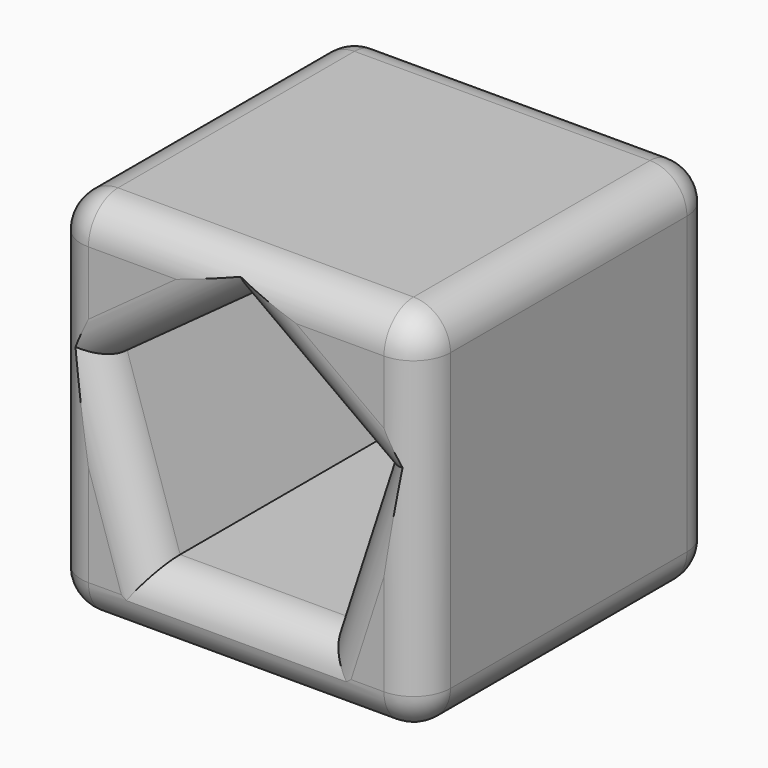
from build123d import *

# Parameters (mm, degrees)
F0_W          = 100
F0_H          = 100
F1_DEPTH      = 100
F3_DEPTH      = 134.3
F4_T1_DEPTH   = 80
F4_T3_DEPTH   = 80
F4_T5_DEPTH   = 80
F4_S9_W       = 10
F4_S9_H       = 10
F4_T10_DEPTH  = 10
F4_S15_W      = 10
F4_S15_H      = 10
F4_T16_DEPTH  = 10
F4_S21_W      = 10
F4_S21_H      = 10
F4_T22_DEPTH  = 10
F4_S27_W      = 10
F4_S27_H      = 10
F4_T28_DEPTH  = 10
F4_S33_W      = 10
F4_S33_H      = 10
F4_T34_DEPTH  = 10
F4_S39_W      = 10
F4_S39_H      = 10
F4_T40_DEPTH  = 10
F4_S45_W      = 10
F4_S45_H      = 10
F4_T46_DEPTH  = 10
F4_S51_W      = 10
F4_S51_H      = 10
F4_T52_DEPTH  = 10
F4_T58_DEPTH  = 96.3793887771
F4_T64_DEPTH  = 96.3793887771
F4_T70_DEPTH  = 96.3793887771
F4_T76_DEPTH  = 96.3793887771
F4_T82_DEPTH  = 96.3793887771
F4_T88_DEPTH  = 96.3793887771
F4_T94_DEPTH  = 96.3793887771
F4_T100_DEPTH = 96.3793887771
F4_T106_DEPTH = 96.3793887771
F4_T112_DEPTH = 96.3793887771
F4_T119_DEPTH = 96.3793887771
F4_T123_DEPTH = 96.3793887771
F4_T130_DEPTH = 96.3793887771
F4_T134_DEPTH = 96.3793887771
F4_T141_DEPTH = 96.3793887771
F4_T145_DEPTH = 96.3793887771
F4_T152_DEPTH = 96.3793887771
F4_T156_DEPTH = 96.3793887771
F4_T163_DEPTH = 96.3793887771
F4_T167_DEPTH = 96.3793887771
F4_T174_DEPTH = 96.3793887771
F4_T178_DEPTH = 96.3793887771
F4_T185_DEPTH = 96.3793887771
F4_T189_DEPTH = 96.3793887771
F4_T196_DEPTH = 96.3793887771
F4_T200_DEPTH = 96.3793887771
F4_T207_DEPTH = 96.3793887771
F4_T211_DEPTH = 96.3793887771
F4_T218_DEPTH = 96.3793887771
F4_T222_DEPTH = 96.3793887771


# Not quite as in the source:
# - a fillet or chamfer that OpenCascade refuses, or shapes differently, is made with other operations: its cross-section is extruded or revolved along the edge and cut away or added


with BuildPart() as f1:
    # F0 (on Front) → F1 (new body)
    with BuildSketch(Plane.XZ):
        Rectangle(F0_W, F0_H)
    extrude(amount=F1_DEPTH)

    # F2 (on face) → F3 (cut)
    with BuildSketch(Plane.XZ.offset(100)):
        Polygon((37.5217137094, 12.1915438206), (0, 39.4526645541), (-37.5217137094, 12.1915438206), (-23.1896943886, -31.9178760977), (23.1896943886, -31.9178760977), align=None)
    extrude(amount=-F3_DEPTH, mode=Mode.SUBTRACT)

    # F4: fillet of radius 10 on 22 edges, made by hand

    # F4_s2 → F4_t1 (cut)
    with BuildSketch(Plane.XZ.offset(10)):
        with BuildLine():
            ThreePointArc((50, -40), (47.0710678119, -47.0710678119), (40, -50))
            Line((40, -50), (50, -50))
            Line((50, -50), (50, -40))
        make_face()
        with BuildLine():
            ThreePointArc((50, 40), (47.0710678119, 47.0710678119), (40, 50))
            Line((40, 50), (50, 50))
            Line((50, 50), (50, 40))
        make_face()
        with BuildLine():
            ThreePointArc((-40, 50), (-47.0710678119, 47.0710678119), (-50, 40))
            Line((-50, 40), (-50, 50))
            Line((-50, 50), (-40, 50))
        make_face()
        with BuildLine():
            ThreePointArc((-40, -50), (-47.0710678119, -47.0710678119), (-50, -40))
            Line((-50, -40), (-50, -50))
            Line((-50, -50), (-40, -50))
        make_face()
    extrude(amount=F4_T1_DEPTH, mode=Mode.SUBTRACT)

    # F4_s4 → F4_t3 (cut)
    with BuildSketch(Plane.XY.offset(-40)):
        with BuildLine():
            ThreePointArc((50, -10), (47.0710678119, -2.9289321881), (40, 0))
            Line((40, 0), (50, 0))
            Line((50, 0), (50, -10))
        make_face()
        with BuildLine():
            ThreePointArc((50, -90), (47.0710678119, -97.0710678119), (40, -100))
            Line((40, -100), (50, -100))
            Line((50, -100), (50, -90))
        make_face()
        with BuildLine():
            ThreePointArc((-40, 0), (-47.0710678119, -2.9289321881), (-50, -10))
            Line((-50, -10), (-50, 0))
            Line((-50, 0), (-40, 0))
        make_face()
        with BuildLine():
            ThreePointArc((-40, -100), (-47.0710678119, -97.0710678119), (-50, -90))
            Line((-50, -90), (-50, -100))
            Line((-50, -100), (-40, -100))
        make_face()
    extrude(amount=F4_T3_DEPTH, mode=Mode.SUBTRACT)

    # F4_s6 → F4_t5 (cut)
    with BuildSketch(Plane.YZ.offset(-40)):
        with BuildLine():
            ThreePointArc((-10, 50), (-2.9289321881, 47.0710678119), (0, 40))
            Line((0, 40), (0, 50))
            Line((0, 50), (-10, 50))
        make_face()
        with BuildLine():
            ThreePointArc((-90, 50), (-97.0710678119, 47.0710678119), (-100, 40))
            Line((-100, 40), (-100, 50))
            Line((-100, 50), (-90, 50))
        make_face()
        with BuildLine():
            ThreePointArc((-10, -50), (-2.9289321881, -47.0710678119), (0, -40))
            Line((0, -40), (0, -50))
            Line((0, -50), (-10, -50))
        make_face()
        with BuildLine():
            ThreePointArc((-90, -50), (-97.0710678119, -47.0710678119), (-100, -40))
            Line((-100, -40), (-100, -50))
            Line((-100, -50), (-90, -50))
        make_face()
    extrude(amount=F4_T5_DEPTH, mode=Mode.SUBTRACT)


with BuildPart() as f4_tool8:
    # F4_s9 → F4_t10 (new body)
    with BuildSketch(Plane.YZ.offset(40)):
        with Locations((-5, -45)):
            Rectangle(F4_S9_W, F4_S9_H)
    extrude(amount=F4_T10_DEPTH)

    # F4_s11 → F4_t12 (revolve, cut)
    with BuildSketch(Plane(origin=(40, -10, -40), x_dir=(0, -0.7071067812, 0.7071067812), z_dir=(0, 0.7071067812, 0.7071067812))):
        with BuildLine():
            ThreePointArc((0, -10), (10, 0), (0, 10))
            Line((0, 10), (0, -10))
        make_face()
    revolve(axis=Axis((40, -10, -40), (1, 0, 0)), mode=Mode.SUBTRACT)


with BuildPart() as f1_1:
    add(f1.part)

    # F4_t7: cut F4_tool8
    add(f4_tool8.part, mode=Mode.SUBTRACT)


with BuildPart() as f4_tool14:
    # F4_s15 → F4_t16 (new body)
    with BuildSketch(Plane.YZ.offset(40)):
        with Locations((-95, -45)):
            Rectangle(F4_S15_W, F4_S15_H)
    extrude(amount=F4_T16_DEPTH)

    # F4_s17 → F4_t18 (revolve, cut)
    with BuildSketch(Plane(origin=(40, -90, -40), x_dir=(0, 0.7071067812, 0.7071067812), z_dir=(0, 0.7071067812, -0.7071067812))):
        with BuildLine():
            ThreePointArc((0, -10), (10, 0), (0, 10))
            Line((0, 10), (0, -10))
        make_face()
    revolve(axis=Axis((40, -90, -40), (1, 0, 0)), mode=Mode.SUBTRACT)


with BuildPart() as f1_2:
    add(f1_1.part)

    # F4_t13: cut F4_tool14
    add(f4_tool14.part, mode=Mode.SUBTRACT)


with BuildPart() as f4_tool20:
    # F4_s21 → F4_t22 (new body)
    with BuildSketch(Plane.YZ.offset(40)):
        with Locations((-5, 45)):
            Rectangle(F4_S21_W, F4_S21_H)
    extrude(amount=F4_T22_DEPTH)

    # F4_s23 → F4_t24 (revolve, cut)
    with BuildSketch(Plane(origin=(40, -10, 40), x_dir=(0, -0.7071067812, -0.7071067812), z_dir=(0, -0.7071067812, 0.7071067812))):
        with BuildLine():
            ThreePointArc((0, -10), (10, 0), (0, 10))
            Line((0, 10), (0, -10))
        make_face()
    revolve(axis=Axis((40, -10, 40), (1, 0, 0)), mode=Mode.SUBTRACT)


with BuildPart() as f1_3:
    add(f1_2.part)

    # F4_t19: cut F4_tool20
    add(f4_tool20.part, mode=Mode.SUBTRACT)


with BuildPart() as f4_tool26:
    # F4_s27 → F4_t28 (new body)
    with BuildSketch(Plane.YZ.offset(40)):
        with Locations((-95, 45)):
            Rectangle(F4_S27_W, F4_S27_H)
    extrude(amount=F4_T28_DEPTH)

    # F4_s29 → F4_t30 (revolve, cut)
    with BuildSketch(Plane(origin=(40, -90, 40), x_dir=(0, 0.7071067812, -0.7071067812), z_dir=(0, -0.7071067812, -0.7071067812))):
        with BuildLine():
            ThreePointArc((0, -10), (10, 0), (0, 10))
            Line((0, 10), (0, -10))
        make_face()
    revolve(axis=Axis((40, -90, 40), (1, 0, 0)), mode=Mode.SUBTRACT)


with BuildPart() as f1_4:
    add(f1_3.part)

    # F4_t25: cut F4_tool26
    add(f4_tool26.part, mode=Mode.SUBTRACT)


with BuildPart() as f4_tool32:
    # F4_s33 → F4_t34 (new body)
    with BuildSketch(Plane.XY.offset(40)):
        with Locations((-45, -5)):
            Rectangle(F4_S33_W, F4_S33_H)
    extrude(amount=F4_T34_DEPTH)

    # F4_s35 → F4_t36 (revolve, cut)
    with BuildSketch(Plane(origin=(-40, -10, 40), x_dir=(0.7071067812, -0.7071067812, 0), z_dir=(-0.7071067812, -0.7071067812, 0))):
        with BuildLine():
            ThreePointArc((0, -10), (10, 0), (0, 10))
            Line((0, 10), (0, -10))
        make_face()
    revolve(axis=Axis((-40, -10, 40), (0, 0, 1)), mode=Mode.SUBTRACT)


with BuildPart() as f1_5:
    add(f1_4.part)

    # F4_t31: cut F4_tool32
    add(f4_tool32.part, mode=Mode.SUBTRACT)


with BuildPart() as f4_tool38:
    # F4_s39 → F4_t40 (new body)
    with BuildSketch(Plane.XY.offset(40)):
        with Locations((-45, -95)):
            Rectangle(F4_S39_W, F4_S39_H)
    extrude(amount=F4_T40_DEPTH)

    # F4_s41 → F4_t42 (revolve, cut)
    with BuildSketch(Plane(origin=(-40, -90, 40), x_dir=(0.7071067812, 0.7071067812, 0), z_dir=(0.7071067812, -0.7071067812, 0))):
        with BuildLine():
            ThreePointArc((0, -10), (10, 0), (0, 10))
            Line((0, 10), (0, -10))
        make_face()
    revolve(axis=Axis((-40, -90, 40), (0, 0, 1)), mode=Mode.SUBTRACT)


with BuildPart() as f1_6:
    add(f1_5.part)

    # F4_t37: cut F4_tool38
    add(f4_tool38.part, mode=Mode.SUBTRACT)


with BuildPart() as f4_tool44:
    # F4_s45 → F4_t46 (new body)
    with BuildSketch(Plane.XY.offset(-40)):
        with Locations((-45, -5)):
            Rectangle(F4_S45_W, F4_S45_H)
    extrude(amount=-F4_T46_DEPTH)

    # F4_s47 → F4_t48 (revolve, cut)
    with BuildSketch(Plane(origin=(-40, -10, -40), x_dir=(0.7071067812, -0.7071067812, 0), z_dir=(0.7071067812, 0.7071067812, 0))):
        with BuildLine():
            ThreePointArc((0, -10), (10, 0), (0, 10))
            Line((0, 10), (0, -10))
        make_face()
    revolve(axis=Axis((-40, -10, -40), (0, 0, -1)), mode=Mode.SUBTRACT)


with BuildPart() as f1_7:
    add(f1_6.part)

    # F4_t43: cut F4_tool44
    add(f4_tool44.part, mode=Mode.SUBTRACT)


with BuildPart() as f4_tool50:
    # F4_s51 → F4_t52 (new body)
    with BuildSketch(Plane.XY.offset(-40)):
        with Locations((-45, -95)):
            Rectangle(F4_S51_W, F4_S51_H)
    extrude(amount=-F4_T52_DEPTH)

    # F4_s53 → F4_t54 (revolve, cut)
    with BuildSketch(Plane(origin=(-40, -90, -40), x_dir=(0.7071067812, 0.7071067812, 0), z_dir=(-0.7071067812, 0.7071067812, 0))):
        with BuildLine():
            ThreePointArc((0, -10), (10, 0), (0, 10))
            Line((0, 10), (0, -10))
        make_face()
    revolve(axis=Axis((-40, -90, -40), (0, 0, -1)), mode=Mode.SUBTRACT)


with BuildPart() as f1_8:
    add(f1_7.part)

    # F4_t49: cut F4_tool50
    add(f4_tool50.part, mode=Mode.SUBTRACT)


with BuildPart() as f4_tool56:
    # F4_s57 → F4_t58 (new body)
    with BuildSketch(Plane(origin=(38.9862817141, 0, -28.3251916741), x_dir=(0, 1, 0), z_dir=(-0.8090169944, 0, 0.5877852523))):
        with BuildLine():
            ThreePointArc((0, -41.9178760977), (-2.9289321881, -34.8468082858), (-10, -31.9178760977))
            Line((-10, -31.9178760977), (0, -31.9178760977))
            Line((0, -31.9178760977), (0, -41.9178760977))
        make_face()
    extrude(amount=F4_T58_DEPTH)

    split(bisect_by=Plane(origin=(-18.7608568547, 0, 25.8221041874), x_dir=(0, 1, 0), z_dir=(0.5877852523, 0, -0.8090169944)), keep=Keep.TOP)

    split(bisect_by=Plane(origin=(30.355704049, 0, -9.8631661385), x_dir=(0, 1, 0), z_dir=(-0.9510565163, 0, 0.3090169944)), keep=Keep.TOP)


with BuildPart() as f1_9:
    add(f1_8.part)

    # F4_t55: cut F4_tool56
    add(f4_tool56.part, mode=Mode.SUBTRACT)


with BuildPart() as f4_tool62:
    # F4_s63 → F4_t64 (new body)
    with BuildSketch(Plane(origin=(38.9862817141, 0, 28.3251916741), x_dir=(0, 1, 0), z_dir=(-0.8090169944, 0, -0.5877852523))):
        with BuildLine():
            ThreePointArc((0, -41.9178760977), (-2.9289321881, -34.8468082858), (-10, -31.9178760977))
            Line((-10, -31.9178760977), (0, -31.9178760977))
            Line((0, -31.9178760977), (0, -41.9178760977))
        make_face()
    extrude(amount=F4_T64_DEPTH)

    split(bisect_by=Plane(origin=(18.7608568547, 0, 25.8221041874), x_dir=(0, 1, 0), z_dir=(-0.5877852523, 0, -0.8090169944)), keep=Keep.TOP)

    split(bisect_by=Plane(origin=(-30.355704049, 0, -9.8631661385), x_dir=(0, 1, 0), z_dir=(0.9510565163, 0, 0.3090169944)), keep=Keep.TOP)


with BuildPart() as f1_10:
    add(f1_9.part)

    # F4_t61: cut F4_tool62
    add(f4_tool62.part, mode=Mode.SUBTRACT)


with BuildPart() as f4_tool68:
    # F4_s69 → F4_t70 (new body)
    with BuildSketch(Plane(origin=(-14.8914345198, 0, 45.8311228665), x_dir=(0, 1, 0), z_dir=(0.3090169944, 0, -0.9510565163))):
        with BuildLine():
            ThreePointArc((0, -41.9178760977), (-2.9289321881, -34.8468082858), (-10, -31.9178760977))
            Line((-10, -31.9178760977), (0, -31.9178760977))
            Line((0, -31.9178760977), (0, -41.9178760977))
        make_face()
    extrude(amount=F4_T70_DEPTH)

    split(bisect_by=Plane(origin=(-18.7608568547, 0, 25.8221041874), x_dir=(0, 1, 0), z_dir=(0.5877852523, 0, -0.8090169944)), keep=Keep.TOP)

    split(bisect_by=Plane.XY.offset(-31.9178760977), keep=Keep.TOP)


with BuildPart() as f1_11:
    add(f1_10.part)

    # F4_t67: cut F4_tool68
    add(f4_tool68.part, mode=Mode.SUBTRACT)


with BuildPart() as f4_tool74:
    # F4_s75 → F4_t76 (new body)
    with BuildSketch(Plane.YZ.offset(-48.1896943886)):
        with BuildLine():
            ThreePointArc((0, -41.9178760977), (-2.9289321881, -34.8468082858), (-10, -31.9178760977))
            Line((-10, -31.9178760977), (0, -31.9178760977))
            Line((0, -31.9178760977), (0, -41.9178760977))
        make_face()
    extrude(amount=F4_T76_DEPTH)

    split(bisect_by=Plane(origin=(-30.355704049, 0, -9.8631661385), x_dir=(0, 1, 0), z_dir=(0.9510565163, 0, 0.3090169944)), keep=Keep.TOP)

    split(bisect_by=Plane(origin=(30.355704049, 0, -9.8631661385), x_dir=(0, 1, 0), z_dir=(-0.9510565163, 0, 0.3090169944)), keep=Keep.TOP)


with BuildPart() as f1_12:
    add(f1_11.part)

    # F4_t73: cut F4_tool74
    add(f4_tool74.part, mode=Mode.SUBTRACT)


with BuildPart() as f4_tool80:
    # F4_s81 → F4_t82 (new body)
    with BuildSketch(Plane(origin=(-14.8914345198, 0, -45.8311228665), x_dir=(0, 1, 0), z_dir=(0.3090169944, 0, 0.9510565163))):
        with BuildLine():
            ThreePointArc((0, -41.9178760977), (-2.9289321881, -34.8468082858), (-10, -31.9178760977))
            Line((-10, -31.9178760977), (0, -31.9178760977))
            Line((0, -31.9178760977), (0, -41.9178760977))
        make_face()
    extrude(amount=F4_T82_DEPTH)

    split(bisect_by=Plane(origin=(18.7608568547, 0, 25.8221041874), x_dir=(0, 1, 0), z_dir=(-0.5877852523, 0, -0.8090169944)), keep=Keep.TOP)

    split(bisect_by=Plane.XY.offset(-31.9178760977), keep=Keep.TOP)


with BuildPart() as f1_13:
    add(f1_12.part)

    # F4_t79: cut F4_tool80
    add(f4_tool80.part, mode=Mode.SUBTRACT)


with BuildPart() as f4_tool86:
    # F4_s87 → F4_t88 (new body)
    with BuildSketch(Plane(origin=(38.9862817141, 0, -28.3251916741), x_dir=(0, 1, 0), z_dir=(-0.8090169944, 0, 0.5877852523))):
        with BuildLine():
            ThreePointArc((-100, -41.9178760977), (-97.0710678119, -34.8468082858), (-90, -31.9178760977))
            Line((-90, -31.9178760977), (-100, -31.9178760977))
            Line((-100, -31.9178760977), (-100, -41.9178760977))
        make_face()
    extrude(amount=F4_T88_DEPTH)

    split(bisect_by=Plane(origin=(-18.7608568547, 0, 25.8221041874), x_dir=(0, 1, 0), z_dir=(0.5877852523, 0, -0.8090169944)), keep=Keep.TOP)

    split(bisect_by=Plane(origin=(30.355704049, 0, -9.8631661385), x_dir=(0, 1, 0), z_dir=(-0.9510565163, 0, 0.3090169944)), keep=Keep.TOP)


with BuildPart() as f1_14:
    add(f1_13.part)

    # F4_t85: cut F4_tool86
    add(f4_tool86.part, mode=Mode.SUBTRACT)


with BuildPart() as f4_tool92:
    # F4_s93 → F4_t94 (new body)
    with BuildSketch(Plane(origin=(38.9862817141, 0, 28.3251916741), x_dir=(0, 1, 0), z_dir=(-0.8090169944, 0, -0.5877852523))):
        with BuildLine():
            ThreePointArc((-100, -41.9178760977), (-97.0710678119, -34.8468082858), (-90, -31.9178760977))
            Line((-90, -31.9178760977), (-100, -31.9178760977))
            Line((-100, -31.9178760977), (-100, -41.9178760977))
        make_face()
    extrude(amount=F4_T94_DEPTH)

    split(bisect_by=Plane(origin=(18.7608568547, 0, 25.8221041874), x_dir=(0, 1, 0), z_dir=(-0.5877852523, 0, -0.8090169944)), keep=Keep.TOP)

    split(bisect_by=Plane(origin=(-30.355704049, 0, -9.8631661385), x_dir=(0, 1, 0), z_dir=(0.9510565163, 0, 0.3090169944)), keep=Keep.TOP)


with BuildPart() as f1_15:
    add(f1_14.part)

    # F4_t91: cut F4_tool92
    add(f4_tool92.part, mode=Mode.SUBTRACT)


with BuildPart() as f4_tool98:
    # F4_s99 → F4_t100 (new body)
    with BuildSketch(Plane(origin=(-14.8914345198, 0, 45.8311228665), x_dir=(0, 1, 0), z_dir=(0.3090169944, 0, -0.9510565163))):
        with BuildLine():
            ThreePointArc((-100, -41.9178760977), (-97.0710678119, -34.8468082858), (-90, -31.9178760977))
            Line((-90, -31.9178760977), (-100, -31.9178760977))
            Line((-100, -31.9178760977), (-100, -41.9178760977))
        make_face()
    extrude(amount=F4_T100_DEPTH)

    split(bisect_by=Plane(origin=(-18.7608568547, 0, 25.8221041874), x_dir=(0, 1, 0), z_dir=(0.5877852523, 0, -0.8090169944)), keep=Keep.TOP)

    split(bisect_by=Plane.XY.offset(-31.9178760977), keep=Keep.TOP)


with BuildPart() as f1_16:
    add(f1_15.part)

    # F4_t97: cut F4_tool98
    add(f4_tool98.part, mode=Mode.SUBTRACT)


with BuildPart() as f4_tool104:
    # F4_s105 → F4_t106 (new body)
    with BuildSketch(Plane.YZ.offset(-48.1896943886)):
        with BuildLine():
            ThreePointArc((-100, -41.9178760977), (-97.0710678119, -34.8468082858), (-90, -31.9178760977))
            Line((-90, -31.9178760977), (-100, -31.9178760977))
            Line((-100, -31.9178760977), (-100, -41.9178760977))
        make_face()
    extrude(amount=F4_T106_DEPTH)

    split(bisect_by=Plane(origin=(-30.355704049, 0, -9.8631661385), x_dir=(0, 1, 0), z_dir=(0.9510565163, 0, 0.3090169944)), keep=Keep.TOP)

    split(bisect_by=Plane(origin=(30.355704049, 0, -9.8631661385), x_dir=(0, 1, 0), z_dir=(-0.9510565163, 0, 0.3090169944)), keep=Keep.TOP)


with BuildPart() as f1_17:
    add(f1_16.part)

    # F4_t103: cut F4_tool104
    add(f4_tool104.part, mode=Mode.SUBTRACT)


with BuildPart() as f4_tool110:
    # F4_s111 → F4_t112 (new body)
    with BuildSketch(Plane(origin=(-14.8914345198, 0, -45.8311228665), x_dir=(0, 1, 0), z_dir=(0.3090169944, 0, 0.9510565163))):
        with BuildLine():
            ThreePointArc((-100, -41.9178760977), (-97.0710678119, -34.8468082858), (-90, -31.9178760977))
            Line((-90, -31.9178760977), (-100, -31.9178760977))
            Line((-100, -31.9178760977), (-100, -41.9178760977))
        make_face()
    extrude(amount=F4_T112_DEPTH)

    split(bisect_by=Plane(origin=(18.7608568547, 0, 25.8221041874), x_dir=(0, 1, 0), z_dir=(-0.5877852523, 0, -0.8090169944)), keep=Keep.TOP)

    split(bisect_by=Plane.XY.offset(-31.9178760977), keep=Keep.TOP)


with BuildPart() as f1_18:
    add(f1_17.part)

    # F4_t109: cut F4_tool110
    add(f4_tool110.part, mode=Mode.SUBTRACT)


with BuildPart() as f4_tool117:
    # F4_s118 → F4_t119 (new body)
    with BuildSketch(Plane(origin=(38.9862817141, 0, -28.3251916741), x_dir=(0, 1, 0), z_dir=(-0.8090169944, 0, 0.5877852523))):
        with BuildLine():
            ThreePointArc((0, -41.9178760977), (-2.9289321881, -34.8468082858), (-10, -31.9178760977))
            Line((-10, -31.9178760977), (0, -31.9178760977))
            Line((0, -31.9178760977), (0, -41.9178760977))
        make_face()
    extrude(amount=F4_T119_DEPTH)

    split(bisect_by=Plane(origin=(30.355704049, 0, -9.8631661385), x_dir=(0, 1, 0), z_dir=(0.9510565163, 0, -0.3090169944)), keep=Keep.TOP)


with BuildPart() as f4_tool121:
    # F4_s122 → F4_t123 (new body)
    with BuildSketch(Plane(origin=(-14.8914345198, 0, -45.8311228665), x_dir=(0, 1, 0), z_dir=(0.3090169944, 0, 0.9510565163))):
        with BuildLine():
            ThreePointArc((0, -41.9178760977), (-2.9289321881, -34.8468082858), (-10, -31.9178760977))
            Line((-10, -31.9178760977), (0, -31.9178760977))
            Line((0, -31.9178760977), (0, -41.9178760977))
        make_face()
    extrude(amount=F4_T123_DEPTH)

    split(bisect_by=Plane(origin=(18.7608568547, 0, 25.8221041874), x_dir=(0, 1, 0), z_dir=(0.5877852523, 0, 0.8090169944)), keep=Keep.TOP)


with BuildPart() as f4_tool117_1:
    add(f4_tool117.part)

    # F4_t125: intersect F4_tool121
    add(f4_tool121.part, mode=Mode.INTERSECT)


with BuildPart() as f1_19:
    add(f1_18.part)

    # F4_t115: cut F4_tool117
    add(f4_tool117_1.part, mode=Mode.SUBTRACT)


with BuildPart() as f4_tool128:
    # F4_s129 → F4_t130 (new body)
    with BuildSketch(Plane(origin=(38.9862817141, 0, -28.3251916741), x_dir=(0, 1, 0), z_dir=(-0.8090169944, 0, 0.5877852523))):
        with BuildLine():
            ThreePointArc((0, -41.9178760977), (-2.9289321881, -34.8468082858), (-10, -31.9178760977))
            Line((-10, -31.9178760977), (0, -31.9178760977))
            Line((0, -31.9178760977), (0, -41.9178760977))
        make_face()
    extrude(amount=F4_T130_DEPTH)

    split(bisect_by=Plane(origin=(-18.7608568547, 0, 25.8221041874), x_dir=(0, 1, 0), z_dir=(-0.5877852523, 0, 0.8090169944)), keep=Keep.TOP)


with BuildPart() as f4_tool132:
    # F4_s133 → F4_t134 (new body)
    with BuildSketch(Plane(origin=(38.9862817141, 0, 28.3251916741), x_dir=(0, 1, 0), z_dir=(-0.8090169944, 0, -0.5877852523))):
        with BuildLine():
            ThreePointArc((0, -41.9178760977), (-2.9289321881, -34.8468082858), (-10, -31.9178760977))
            Line((-10, -31.9178760977), (0, -31.9178760977))
            Line((0, -31.9178760977), (0, -41.9178760977))
        make_face()
    extrude(amount=F4_T134_DEPTH)

    split(bisect_by=Plane(origin=(18.7608568547, 0, 25.8221041874), x_dir=(0, 1, 0), z_dir=(0.5877852523, 0, 0.8090169944)), keep=Keep.TOP)


with BuildPart() as f4_tool128_1:
    add(f4_tool128.part)

    # F4_t136: intersect F4_tool132
    add(f4_tool132.part, mode=Mode.INTERSECT)


with BuildPart() as f1_20:
    add(f1_19.part)

    # F4_t126: cut F4_tool128
    add(f4_tool128_1.part, mode=Mode.SUBTRACT)


with BuildPart() as f4_tool139:
    # F4_s140 → F4_t141 (new body)
    with BuildSketch(Plane(origin=(38.9862817141, 0, 28.3251916741), x_dir=(0, 1, 0), z_dir=(-0.8090169944, 0, -0.5877852523))):
        with BuildLine():
            ThreePointArc((0, -41.9178760977), (-2.9289321881, -34.8468082858), (-10, -31.9178760977))
            Line((-10, -31.9178760977), (0, -31.9178760977))
            Line((0, -31.9178760977), (0, -41.9178760977))
        make_face()
    extrude(amount=F4_T141_DEPTH)

    split(bisect_by=Plane(origin=(-30.355704049, 0, -9.8631661385), x_dir=(0, 1, 0), z_dir=(-0.9510565163, 0, -0.3090169944)), keep=Keep.TOP)


with BuildPart() as f4_tool143:
    # F4_s144 → F4_t145 (new body)
    with BuildSketch(Plane(origin=(-14.8914345198, 0, 45.8311228665), x_dir=(0, 1, 0), z_dir=(0.3090169944, 0, -0.9510565163))):
        with BuildLine():
            ThreePointArc((0, -41.9178760977), (-2.9289321881, -34.8468082858), (-10, -31.9178760977))
            Line((-10, -31.9178760977), (0, -31.9178760977))
            Line((0, -31.9178760977), (0, -41.9178760977))
        make_face()
    extrude(amount=F4_T145_DEPTH)

    split(bisect_by=Plane(origin=(-18.7608568547, 0, 25.8221041874), x_dir=(0, 1, 0), z_dir=(-0.5877852523, 0, 0.8090169944)), keep=Keep.TOP)


with BuildPart() as f4_tool139_1:
    add(f4_tool139.part)

    # F4_t147: intersect F4_tool143
    add(f4_tool143.part, mode=Mode.INTERSECT)


with BuildPart() as f1_21:
    add(f1_20.part)

    # F4_t137: cut F4_tool139
    add(f4_tool139_1.part, mode=Mode.SUBTRACT)


with BuildPart() as f4_tool150:
    # F4_s151 → F4_t152 (new body)
    with BuildSketch(Plane(origin=(-14.8914345198, 0, 45.8311228665), x_dir=(0, 1, 0), z_dir=(0.3090169944, 0, -0.9510565163))):
        with BuildLine():
            ThreePointArc((0, -41.9178760977), (-2.9289321881, -34.8468082858), (-10, -31.9178760977))
            Line((-10, -31.9178760977), (0, -31.9178760977))
            Line((0, -31.9178760977), (0, -41.9178760977))
        make_face()
    extrude(amount=F4_T152_DEPTH)

    split(bisect_by=Plane.XY.offset(-31.9178760977), keep=Keep.BOTTOM)


with BuildPart() as f4_tool154:
    # F4_s155 → F4_t156 (new body)
    with BuildSketch(Plane.YZ.offset(-48.1896943886)):
        with BuildLine():
            ThreePointArc((0, -41.9178760977), (-2.9289321881, -34.8468082858), (-10, -31.9178760977))
            Line((-10, -31.9178760977), (0, -31.9178760977))
            Line((0, -31.9178760977), (0, -41.9178760977))
        make_face()
    extrude(amount=F4_T156_DEPTH)

    split(bisect_by=Plane(origin=(-30.355704049, 0, -9.8631661385), x_dir=(0, 1, 0), z_dir=(-0.9510565163, 0, -0.3090169944)), keep=Keep.TOP)


with BuildPart() as f4_tool150_1:
    add(f4_tool150.part)

    # F4_t158: intersect F4_tool154
    add(f4_tool154.part, mode=Mode.INTERSECT)


with BuildPart() as f1_22:
    add(f1_21.part)

    # F4_t148: cut F4_tool150
    add(f4_tool150_1.part, mode=Mode.SUBTRACT)


with BuildPart() as f4_tool161:
    # F4_s162 → F4_t163 (new body)
    with BuildSketch(Plane.YZ.offset(-48.1896943886)):
        with BuildLine():
            ThreePointArc((0, -41.9178760977), (-2.9289321881, -34.8468082858), (-10, -31.9178760977))
            Line((-10, -31.9178760977), (0, -31.9178760977))
            Line((0, -31.9178760977), (0, -41.9178760977))
        make_face()
    extrude(amount=F4_T163_DEPTH)

    split(bisect_by=Plane(origin=(30.355704049, 0, -9.8631661385), x_dir=(0, 1, 0), z_dir=(0.9510565163, 0, -0.3090169944)), keep=Keep.TOP)


with BuildPart() as f4_tool165:
    # F4_s166 → F4_t167 (new body)
    with BuildSketch(Plane(origin=(-14.8914345198, 0, -45.8311228665), x_dir=(0, 1, 0), z_dir=(0.3090169944, 0, 0.9510565163))):
        with BuildLine():
            ThreePointArc((0, -41.9178760977), (-2.9289321881, -34.8468082858), (-10, -31.9178760977))
            Line((-10, -31.9178760977), (0, -31.9178760977))
            Line((0, -31.9178760977), (0, -41.9178760977))
        make_face()
    extrude(amount=F4_T167_DEPTH)

    split(bisect_by=Plane.XY.offset(-31.9178760977), keep=Keep.BOTTOM)


with BuildPart() as f4_tool161_1:
    add(f4_tool161.part)

    # F4_t169: intersect F4_tool165
    add(f4_tool165.part, mode=Mode.INTERSECT)


with BuildPart() as f1_23:
    add(f1_22.part)

    # F4_t159: cut F4_tool161
    add(f4_tool161_1.part, mode=Mode.SUBTRACT)


with BuildPart() as f4_tool172:
    # F4_s173 → F4_t174 (new body)
    with BuildSketch(Plane(origin=(38.9862817141, 0, -28.3251916741), x_dir=(0, 1, 0), z_dir=(-0.8090169944, 0, 0.5877852523))):
        with BuildLine():
            ThreePointArc((-100, -41.9178760977), (-97.0710678119, -34.8468082858), (-90, -31.9178760977))
            Line((-90, -31.9178760977), (-100, -31.9178760977))
            Line((-100, -31.9178760977), (-100, -41.9178760977))
        make_face()
    extrude(amount=F4_T174_DEPTH)

    split(bisect_by=Plane(origin=(30.355704049, 0, -9.8631661385), x_dir=(0, 1, 0), z_dir=(0.9510565163, 0, -0.3090169944)), keep=Keep.TOP)


with BuildPart() as f4_tool176:
    # F4_s177 → F4_t178 (new body)
    with BuildSketch(Plane(origin=(-14.8914345198, 0, -45.8311228665), x_dir=(0, 1, 0), z_dir=(0.3090169944, 0, 0.9510565163))):
        with BuildLine():
            ThreePointArc((-100, -41.9178760977), (-97.0710678119, -34.8468082858), (-90, -31.9178760977))
            Line((-90, -31.9178760977), (-100, -31.9178760977))
            Line((-100, -31.9178760977), (-100, -41.9178760977))
        make_face()
    extrude(amount=F4_T178_DEPTH)

    split(bisect_by=Plane(origin=(18.7608568547, 0, 25.8221041874), x_dir=(0, 1, 0), z_dir=(0.5877852523, 0, 0.8090169944)), keep=Keep.TOP)


with BuildPart() as f4_tool172_1:
    add(f4_tool172.part)

    # F4_t180: intersect F4_tool176
    add(f4_tool176.part, mode=Mode.INTERSECT)


with BuildPart() as f1_24:
    add(f1_23.part)

    # F4_t170: cut F4_tool172
    add(f4_tool172_1.part, mode=Mode.SUBTRACT)


with BuildPart() as f4_tool183:
    # F4_s184 → F4_t185 (new body)
    with BuildSketch(Plane(origin=(38.9862817141, 0, -28.3251916741), x_dir=(0, 1, 0), z_dir=(-0.8090169944, 0, 0.5877852523))):
        with BuildLine():
            ThreePointArc((-100, -41.9178760977), (-97.0710678119, -34.8468082858), (-90, -31.9178760977))
            Line((-90, -31.9178760977), (-100, -31.9178760977))
            Line((-100, -31.9178760977), (-100, -41.9178760977))
        make_face()
    extrude(amount=F4_T185_DEPTH)

    split(bisect_by=Plane(origin=(-18.7608568547, 0, 25.8221041874), x_dir=(0, 1, 0), z_dir=(-0.5877852523, 0, 0.8090169944)), keep=Keep.TOP)


with BuildPart() as f4_tool187:
    # F4_s188 → F4_t189 (new body)
    with BuildSketch(Plane(origin=(38.9862817141, 0, 28.3251916741), x_dir=(0, 1, 0), z_dir=(-0.8090169944, 0, -0.5877852523))):
        with BuildLine():
            ThreePointArc((-100, -41.9178760977), (-97.0710678119, -34.8468082858), (-90, -31.9178760977))
            Line((-90, -31.9178760977), (-100, -31.9178760977))
            Line((-100, -31.9178760977), (-100, -41.9178760977))
        make_face()
    extrude(amount=F4_T189_DEPTH)

    split(bisect_by=Plane(origin=(18.7608568547, 0, 25.8221041874), x_dir=(0, 1, 0), z_dir=(0.5877852523, 0, 0.8090169944)), keep=Keep.TOP)


with BuildPart() as f4_tool183_1:
    add(f4_tool183.part)

    # F4_t191: intersect F4_tool187
    add(f4_tool187.part, mode=Mode.INTERSECT)


with BuildPart() as f1_25:
    add(f1_24.part)

    # F4_t181: cut F4_tool183
    add(f4_tool183_1.part, mode=Mode.SUBTRACT)


with BuildPart() as f4_tool194:
    # F4_s195 → F4_t196 (new body)
    with BuildSketch(Plane(origin=(38.9862817141, 0, 28.3251916741), x_dir=(0, 1, 0), z_dir=(-0.8090169944, 0, -0.5877852523))):
        with BuildLine():
            ThreePointArc((-100, -41.9178760977), (-97.0710678119, -34.8468082858), (-90, -31.9178760977))
            Line((-90, -31.9178760977), (-100, -31.9178760977))
            Line((-100, -31.9178760977), (-100, -41.9178760977))
        make_face()
    extrude(amount=F4_T196_DEPTH)

    split(bisect_by=Plane(origin=(-30.355704049, 0, -9.8631661385), x_dir=(0, 1, 0), z_dir=(-0.9510565163, 0, -0.3090169944)), keep=Keep.TOP)


with BuildPart() as f4_tool198:
    # F4_s199 → F4_t200 (new body)
    with BuildSketch(Plane(origin=(-14.8914345198, 0, 45.8311228665), x_dir=(0, 1, 0), z_dir=(0.3090169944, 0, -0.9510565163))):
        with BuildLine():
            ThreePointArc((-100, -41.9178760977), (-97.0710678119, -34.8468082858), (-90, -31.9178760977))
            Line((-90, -31.9178760977), (-100, -31.9178760977))
            Line((-100, -31.9178760977), (-100, -41.9178760977))
        make_face()
    extrude(amount=F4_T200_DEPTH)

    split(bisect_by=Plane(origin=(-18.7608568547, 0, 25.8221041874), x_dir=(0, 1, 0), z_dir=(-0.5877852523, 0, 0.8090169944)), keep=Keep.TOP)


with BuildPart() as f4_tool194_1:
    add(f4_tool194.part)

    # F4_t202: intersect F4_tool198
    add(f4_tool198.part, mode=Mode.INTERSECT)


with BuildPart() as f1_26:
    add(f1_25.part)

    # F4_t192: cut F4_tool194
    add(f4_tool194_1.part, mode=Mode.SUBTRACT)


with BuildPart() as f4_tool205:
    # F4_s206 → F4_t207 (new body)
    with BuildSketch(Plane(origin=(-14.8914345198, 0, 45.8311228665), x_dir=(0, 1, 0), z_dir=(0.3090169944, 0, -0.9510565163))):
        with BuildLine():
            ThreePointArc((-100, -41.9178760977), (-97.0710678119, -34.8468082858), (-90, -31.9178760977))
            Line((-90, -31.9178760977), (-100, -31.9178760977))
            Line((-100, -31.9178760977), (-100, -41.9178760977))
        make_face()
    extrude(amount=F4_T207_DEPTH)

    split(bisect_by=Plane.XY.offset(-31.9178760977), keep=Keep.BOTTOM)


with BuildPart() as f4_tool209:
    # F4_s210 → F4_t211 (new body)
    with BuildSketch(Plane.YZ.offset(-48.1896943886)):
        with BuildLine():
            ThreePointArc((-100, -41.9178760977), (-97.0710678119, -34.8468082858), (-90, -31.9178760977))
            Line((-90, -31.9178760977), (-100, -31.9178760977))
            Line((-100, -31.9178760977), (-100, -41.9178760977))
        make_face()
    extrude(amount=F4_T211_DEPTH)

    split(bisect_by=Plane(origin=(-30.355704049, 0, -9.8631661385), x_dir=(0, 1, 0), z_dir=(-0.9510565163, 0, -0.3090169944)), keep=Keep.TOP)


with BuildPart() as f4_tool205_1:
    add(f4_tool205.part)

    # F4_t213: intersect F4_tool209
    add(f4_tool209.part, mode=Mode.INTERSECT)


with BuildPart() as f1_27:
    add(f1_26.part)

    # F4_t203: cut F4_tool205
    add(f4_tool205_1.part, mode=Mode.SUBTRACT)


with BuildPart() as f4_tool216:
    # F4_s217 → F4_t218 (new body)
    with BuildSketch(Plane.YZ.offset(-48.1896943886)):
        with BuildLine():
            ThreePointArc((-100, -41.9178760977), (-97.0710678119, -34.8468082858), (-90, -31.9178760977))
            Line((-90, -31.9178760977), (-100, -31.9178760977))
            Line((-100, -31.9178760977), (-100, -41.9178760977))
        make_face()
    extrude(amount=F4_T218_DEPTH)

    split(bisect_by=Plane(origin=(30.355704049, 0, -9.8631661385), x_dir=(0, 1, 0), z_dir=(0.9510565163, 0, -0.3090169944)), keep=Keep.TOP)


with BuildPart() as f4_tool220:
    # F4_s221 → F4_t222 (new body)
    with BuildSketch(Plane(origin=(-14.8914345198, 0, -45.8311228665), x_dir=(0, 1, 0), z_dir=(0.3090169944, 0, 0.9510565163))):
        with BuildLine():
            ThreePointArc((-100, -41.9178760977), (-97.0710678119, -34.8468082858), (-90, -31.9178760977))
            Line((-90, -31.9178760977), (-100, -31.9178760977))
            Line((-100, -31.9178760977), (-100, -41.9178760977))
        make_face()
    extrude(amount=F4_T222_DEPTH)

    split(bisect_by=Plane.XY.offset(-31.9178760977), keep=Keep.BOTTOM)


with BuildPart() as f4_tool216_1:
    add(f4_tool216.part)

    # F4_t224: intersect F4_tool220
    add(f4_tool220.part, mode=Mode.INTERSECT)


with BuildPart() as f1_28:
    add(f1_27.part)

    # F4_t214: cut F4_tool216
    add(f4_tool216_1.part, mode=Mode.SUBTRACT)


solid = f1_28.part
